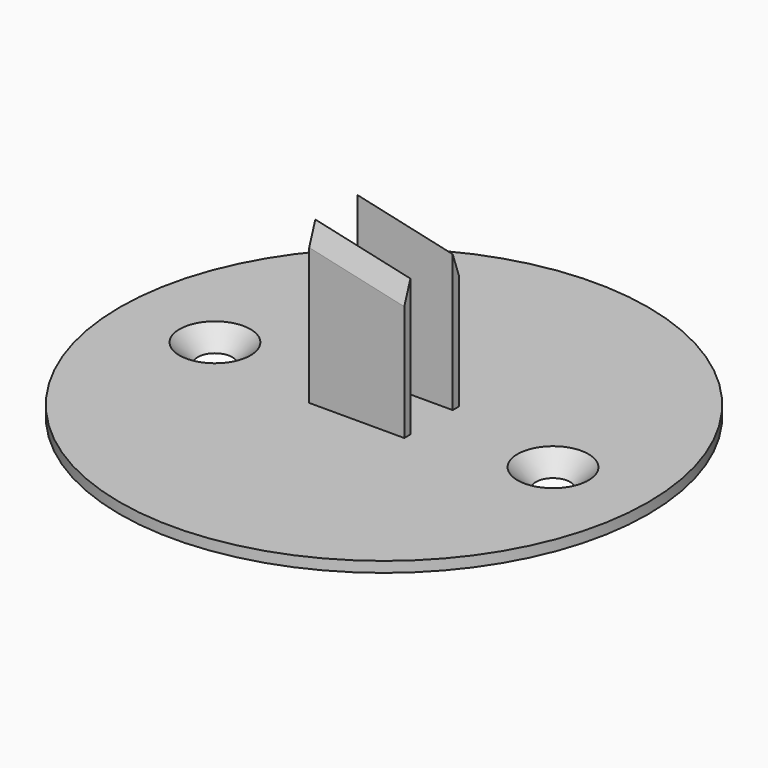
from build123d import *

# Parameters (mm, degrees)
F0_R           = 50
F1_DEPTH       = 2
F3_R           = 10
F4_DEPTH       = 1.5
F5_D           = 6.4
F5_CSINK_D     = 13.44
F5_CSINK_ANGLE = 90
F6_W           = 18
F6_H           = 1.45
F7_DEPTH       = 30
F9_DEPTH       = 25
F10_T1_DEPTH   = 39.192646775


# Not quite as in the source:
# - a fillet or chamfer that OpenCascade refuses, or shapes differently, is made with other operations: its cross-section is extruded or revolved along the edge and cut away or added


with BuildPart() as f1:
    # F0 (on Top) → F1 (new body)
    with BuildSketch(Plane.XY):
        Circle(F0_R)
    extrude(amount=F1_DEPTH)

    # F3 (on face) → F4 (join)
    with BuildSketch(Plane(origin=(0, 0, 0), x_dir=(1, 0, 0), z_dir=(0, 0, -1))):
        with Locations((31.9376476109, 0)):
            Circle(F3_R)
        with Locations((-32.1291722357, 0)):
            Circle(F3_R)
    extrude(amount=F4_DEPTH)

    # F5 (through all)
    with Locations(Plane.XY.offset(2)):
        with Locations((-32, 0), (32, 0)):
            CounterSinkHole(F5_D / 2, F5_CSINK_D / 2, counter_sink_angle=F5_CSINK_ANGLE)

    # F6 (on face) → F7 (join)
    with BuildSketch(Plane.XY.offset(2)):
        with Locations((0, 5.725)):
            Rectangle(F6_W, F6_H)
        with Locations((0, -5.725)):
            Rectangle(F6_W, F6_H)
    extrude(amount=F7_DEPTH)

    # F8 (on face) → F9 (cut)
    with BuildSketch(Plane.XZ.offset(6.45)):
        Polygon((9, 32), (-9, 32), (9, 28), align=None)
    extrude(amount=-F9_DEPTH, mode=Mode.SUBTRACT)

    # F10: chamfer of 4 x 1.4558809371 on 2 edges, made by hand

    # F10_s2 → F10_t1 (cut)
    with BuildSketch(Plane(origin=(-25.4826184945, 0, 5.6628041099), x_dir=(0, 1, 0), z_dir=(0.9761870602, 0, -0.2169304578))):
        Polygon((6.45, 25.2856118055), (4.9941190629, 29.2856118055), (6.45, 29.2856118055), align=None)
        Polygon((-6.45, 25.2856118055), (-4.9941190629, 29.2856118055), (-6.45, 29.2856118055), align=None)
    extrude(amount=F10_T1_DEPTH, mode=Mode.SUBTRACT)


solid = f1.part
